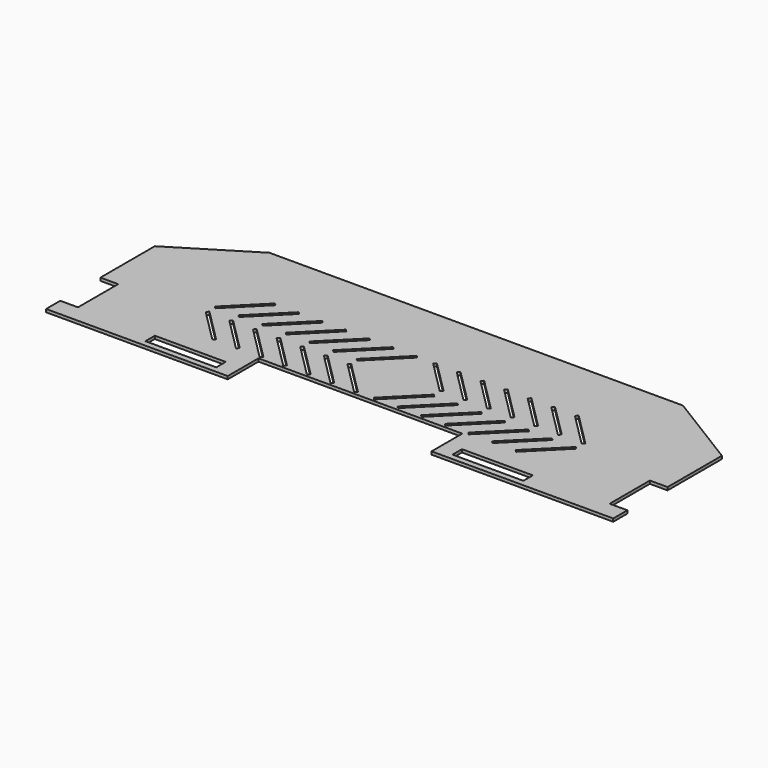
from build123d import *

# Parameters (mm, degrees)
F0_W     = 76.2
F0_H     = 12.7
F1_DEPTH = 3.175
F2_DEPTH = 12.7


# Not quite as in the source:
# - a length typed as a fraction of an inch, garbled in the dataset ("3 / 203.2 mm" for 3/8 in), is restored


with BuildPart() as f1:
    # F0 (on Top) → F1 (new body)
    with BuildSketch(Plane.XY):
        Polygon((285.7501016, -19.0500762), (304.8001016, -19.0500762), (304.8001016, 53.9749238), (222.2501016, 104.7749238), (-222.2500762, 104.7749238), (-304.8000762, 53.9749238), (-304.8000762, -19.0500762), (-285.7500762, -19.0500762), (-285.7500762, -73.0248984), (-304.8000762, -73.0248984), (-304.8000762, -104.7748984), (-109.5373984, -104.7748984), (-109.5373984, -67.4683182), (-244.475254, -67.4683182), (-244.475254, -46.8308182), (-162.5825794541, -46.8308182), (-196.8829692, -12.5304042), (-194.6378124, -10.285222), (-158.7168276, -46.2063846), (-159.3413106539, -46.8308182), (-137.1825794541, -46.8308182), (-171.4829692, -12.5304042), (-169.2378124, -10.285222), (-133.3168276, -46.2063846), (-133.9413106539, -46.8308182), (-111.7825794541, -46.8308182), (-146.0829692, -12.5304042), (-143.8378124, -10.285222), (-107.9168276, -46.2063846), (-108.5413106539, -46.8308182), (-86.3825794541, -46.8308182), (-120.6829692, -12.5304042), (-118.4378124, -10.285222), (-82.5168276, -46.2063846), (-83.1413106539, -46.8308182), (-60.9824096755, -46.8308182), (-95.2829692, -12.5304042), (-93.0378124, -10.285222), (-57.1170054, -46.2063846), (-57.7413895461, -46.8308182), (-35.5824096755, -46.8308182), (-69.8829692, -12.5304042), (-67.6378124, -10.285222), (-31.7170054, -46.2063846), (-32.3413895461, -46.8308182), (-10.1824176969, -46.8308182), (-44.483147, -12.5304042), (-42.2376346, -10.285222), (-6.3170054, -46.2063846), (-6.9413895461, -46.8308182), (11.3860423894, -46.8308182), (10.7618784, -46.2065624), (46.682533, -10.2855776), (48.9280454, -12.5307598), (14.6276231923, -46.8308182), (36.7860423894, -46.8308182), (36.1618784, -46.2065624), (72.082533, -10.2855776), (74.3280454, -12.5307598), (40.0276231923, -46.8308182), (62.1860423894, -46.8308182), (61.5618784, -46.2065624), (97.482533, -10.2855776), (99.7280454, -12.5307598), (65.4276231923, -46.8308182), (87.5860423894, -46.8308182), (86.9618784, -46.2065624), (122.882533, -10.2855776), (125.1280454, -12.5307598), (90.8276231923, -46.8308182), (112.9860423894, -46.8308182), (112.3618784, -46.2065624), (148.282533, -10.2855776), (150.5280454, -12.5307598), (116.2276231923, -46.8308182), (138.3860423894, -46.8308182), (137.7618784, -46.2065624), (173.682533, -10.2855776), (175.9280454, -12.5307598), (141.6276231923, -46.8308182), (163.7860423894, -46.8308182), (163.1618784, -46.2065624), (199.082533, -10.2855776), (201.3280454, -12.5307598), (167.0276231923, -46.8308182), (244.474746, -46.8308182), (244.474746, -67.4683182), (109.5376016, -67.4683182), (109.5376016, -104.7748984), (304.8001016, -104.7748984), (304.8001016, -73.0248984), (285.7501016, -73.0248984), align=None)
        with Locations((-165.052883, -79.3748984)):
            Rectangle(F0_W, F0_H, mode=Mode.SUBTRACT)
        with Locations((165.1001016, -79.3748984)):
            Rectangle(F0_W, F0_H, mode=Mode.SUBTRACT)
        Polygon((-158.7168276, 33.506918), (-194.6378124, -2.4142192), (-196.8829692, -0.1690624), (-160.9620098, 35.7519224), align=None, mode=Mode.SUBTRACT)
        Polygon((-133.3168276, 33.506918), (-169.2378124, -2.4142192), (-171.4829692, -0.1690624), (-135.5620098, 35.7519224), align=None, mode=Mode.SUBTRACT)
        Polygon((-107.9168276, 33.506918), (-143.8378124, -2.4142192), (-146.0829692, -0.1690624), (-110.1620098, 35.7519224), align=None, mode=Mode.SUBTRACT)
        Polygon((-82.5168276, 33.506918), (-118.4378124, -2.4142192), (-120.6829692, -0.1690624), (-84.7620098, 35.7519224), align=None, mode=Mode.SUBTRACT)
        Polygon((-57.1170054, 33.506918), (-93.0378124, -2.4142192), (-95.2829692, -0.1690624), (-59.361832, 35.7519224), align=None, mode=Mode.SUBTRACT)
        Polygon((-31.7170054, 33.506918), (-67.6378124, -2.4142192), (-69.8829692, -0.1690624), (-33.961832, 35.7519224), align=None, mode=Mode.SUBTRACT)
        Polygon((-6.3170054, 33.506918), (-42.2376346, -2.4142192), (-44.483147, -0.1690624), (-8.561832, 35.7519224), align=None, mode=Mode.SUBTRACT)
        Polygon((13.006705, 35.752278), (48.9280454, -0.1687068), (46.682533, -2.413889), (10.7618784, 33.5070958), align=None, mode=Mode.SUBTRACT)
        Polygon((38.406705, 35.752278), (74.3280454, -0.1687068), (72.082533, -2.413889), (36.1618784, 33.5070958), align=None, mode=Mode.SUBTRACT)
        Polygon((63.806705, 35.752278), (99.7280454, -0.1687068), (97.482533, -2.413889), (61.5618784, 33.5070958), align=None, mode=Mode.SUBTRACT)
        Polygon((89.206705, 35.752278), (125.1280454, -0.1687068), (122.882533, -2.413889), (86.9618784, 33.5070958), align=None, mode=Mode.SUBTRACT)
        Polygon((114.606705, 35.752278), (150.5280454, -0.1687068), (148.282533, -2.413889), (112.3618784, 33.5070958), align=None, mode=Mode.SUBTRACT)
        Polygon((140.006705, 35.752278), (175.9280454, -0.1687068), (173.682533, -2.413889), (137.7618784, 33.5070958), align=None, mode=Mode.SUBTRACT)
        Polygon((165.406705, 35.752278), (201.3280454, -0.1687068), (199.082533, -2.413889), (163.1618784, 33.5070958), align=None, mode=Mode.SUBTRACT)
        Polygon((109.5376016, -50.7998984), (109.5376016, -67.4683182), (244.474746, -67.4683182), (244.474746, -46.8308182), (167.0276231923, -46.8308182), (165.406705, -48.4517192), (163.7860423894, -46.8308182), (141.6276231923, -46.8308182), (140.006705, -48.4517192), (138.3860423894, -46.8308182), (116.2276231923, -46.8308182), (114.606705, -48.4517192), (112.9860423894, -46.8308182), (90.8276231923, -46.8308182), (89.206705, -48.4517192), (87.5860423894, -46.8308182), (65.4276231923, -46.8308182), (63.806705, -48.4517192), (62.1860423894, -46.8308182), (40.0276231923, -46.8308182), (38.406705, -48.4517192), (36.7860423894, -46.8308182), (14.6276231923, -46.8308182), (13.006705, -48.4517192), (11.3860423894, -46.8308182), (-6.9413895461, -46.8308182), (-8.561832, -48.451389), (-10.1824176969, -46.8308182), (-32.3413895461, -46.8308182), (-33.961832, -48.451389), (-35.5824096755, -46.8308182), (-57.7413895461, -46.8308182), (-59.361832, -48.451389), (-60.9824096755, -46.8308182), (-83.1413106539, -46.8308182), (-84.7620098, -48.451389), (-86.3825794541, -46.8308182), (-108.5413106539, -46.8308182), (-110.1620098, -48.451389), (-111.7825794541, -46.8308182), (-133.9413106539, -46.8308182), (-135.5620098, -48.451389), (-137.1825794541, -46.8308182), (-159.3413106539, -46.8308182), (-160.9620098, -48.451389), (-162.5825794541, -46.8308182), (-244.475254, -46.8308182), (-244.475254, -67.4683182), (-109.5373984, -67.4683182), (-109.5373984, -50.7998984), align=None)
    extrude(amount=F1_DEPTH)

    # F2 (cut): faces of the model
    f2_faces = [f1.faces().sort_by_distance(p)[0] for p in [
        (-207.1687373, -104.7748984, 1.5875),
        (207.1688516, -104.7748984, 1.5875),
    ]]
    extrude(f2_faces, amount=-F2_DEPTH, mode=Mode.SUBTRACT)


solid = f1.part
